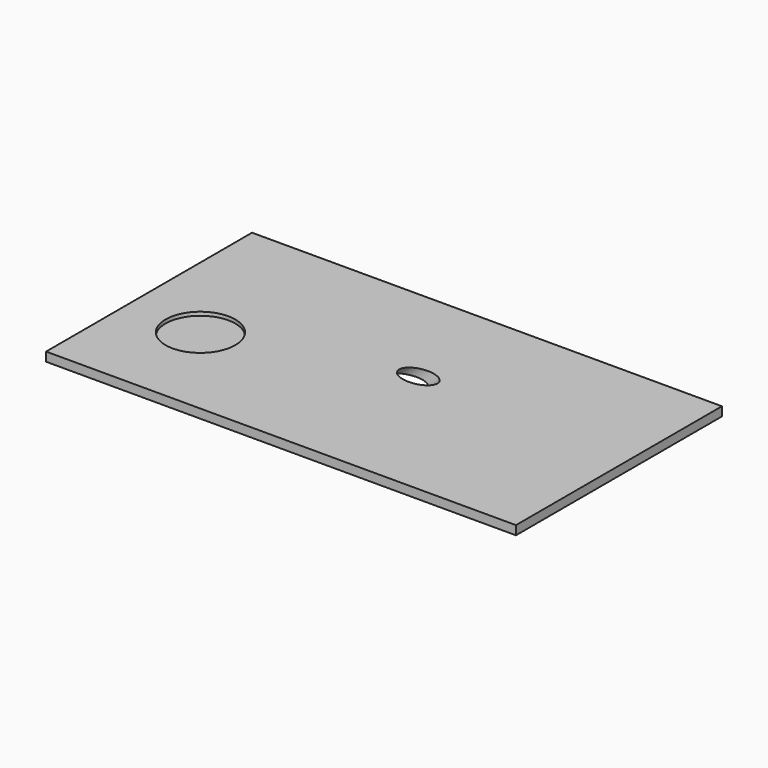
from build123d import *

# Parameters (mm, degrees)
F0_W     = 261.6643384099
F0_H     = 143.3737166226
F1_DEPTH = 5
F2_R     = 19.4105187662
F3_DEPTH = 2
F6_R     = 6.5980928428
F7_DEPTH = 96.0488122602


# Not quite as in the source:
# - a feature of the source that left no trace in its solid (it failed there, or was rolled back) is left out


with BuildPart() as f1:
    # F0 (on Top) → F1 (new body)
    with BuildSketch(Plane.XY):
        with Locations((-11.2871490419, -11.1323576421)):
            Rectangle(F0_W, F0_H)
    extrude(amount=F1_DEPTH)

    # F2 (on face) → F3 (cut)
    with BuildSketch(Plane.XY.offset(5)):
        with Locations((-101.0480299592, -26.7270803452)):
            Circle(F2_R)
    extrude(amount=-F3_DEPTH, mode=Mode.SUBTRACT)


with BuildPart() as f7:
    # F6 (on line) → F7 (new body, through all)
    with BuildSketch(Plane(origin=(41.3091172937, 0, 32.6350144213), x_dir=(0, 1, 0), z_dir=(0.7846743667, 0, 0.6199081692))):
        with Locations((0, 4.5975914841)):
            Circle(F6_R)
    extrude(amount=-F7_DEPTH)


with BuildPart() as f1_1:
    add(f1.part)

    # F8: cut F7
    add(f7.part, mode=Mode.SUBTRACT)


solid = f1_1.part
